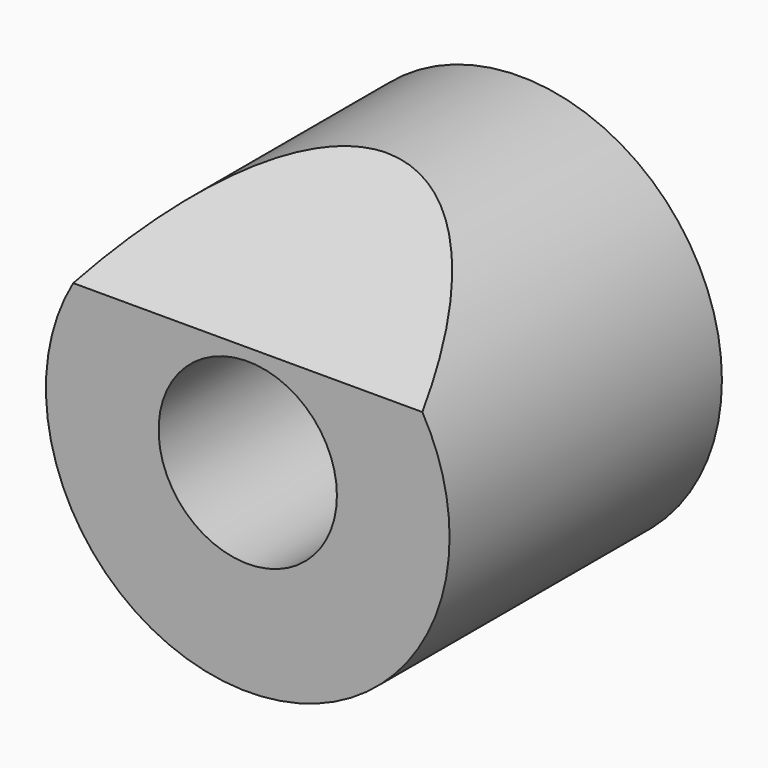
from build123d import *

# Parameters (mm, degrees)
F0_R     = 12.45
F0_R_2   = 5.5
F1_DEPTH = 21
F3_DEPTH = 12.5


with BuildPart() as f1:
    # F0 (on Front) → F1 (new body)
    with BuildSketch(Plane.XZ):
        Circle(F0_R)
        Circle(F0_R_2, mode=Mode.SUBTRACT)
    extrude(amount=F1_DEPTH)

    # F2 (on Right) → F3 (cut, symmetric)
    with BuildSketch(Plane.YZ):
        Polygon((-10.2612849931, 12.45), (-21, 12.45), (-21, 6.25), align=None)
    extrude(amount=F3_DEPTH, both=True, mode=Mode.SUBTRACT)


solid = f1.part
